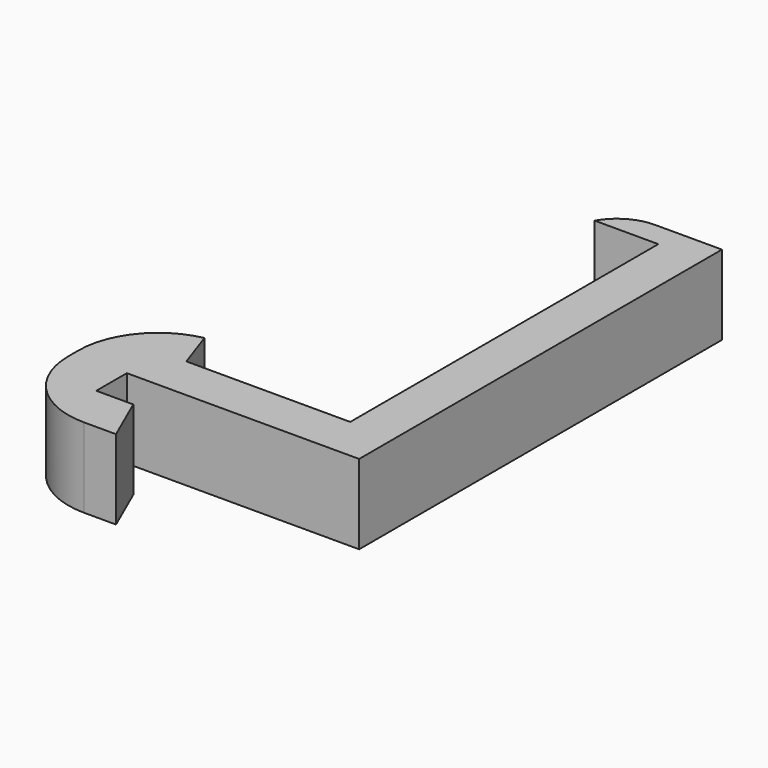
from build123d import *

# Parameters (mm, degrees)
F0_W        = 0.4
F0_H        = 28.4
F1_DEPTH    = 5
F2_T1_DEPTH = 17.9903810568
F3_T1_DEPTH = 29.4948974279
F3_T3_DEPTH = 30


# Not quite as in the source:
# - a fillet or chamfer that OpenCascade refuses, or shapes differently, is made with other operations: its cross-section is extruded or revolved along the edge and cut away or added


with BuildPart() as f1:
    # F0 (on Top) → F1 (new body)
    with BuildSketch(Plane.XY):
        Polygon((-17.5608190332, -5.5), (-10.5608190332, -5.5), (-11.8766345504, -2.5), (-14.2008190332, -2.5), (-14.2008190332, -0.1), (-14.2008190332, 0), (0, 0), (0, 28.4), (-6.4, 28.4), (-6.4, 26.9), (-2.4, 26.9), (-2.4, 2.7), (-12.7, 2.7), (-13.5608190332, 5.2), (-17.5608190332, 5.2), align=None)
        Polygon((-14.2008190332, 0), (-14.2008190332, -0.1), (0.4, -0.1), (0.4, 0), (0, 0), align=None)
        with Locations((0.2, 14.2)):
            Rectangle(F0_W, F0_H)
    extrude(amount=F1_DEPTH)

    # F2: fillet of radius 3 on 1 edges, made by hand

    # F2_s2 → F2_t1 (cut)
    with BuildSketch(Plane.XY.offset(-6.4951905284)):
        with BuildLine():
            ThreePointArc((-3.8019237886, 28.4), (-5.3019237886, 27.9980762114), (-6.4, 26.9))
            Line((-6.4, 26.9), (-6.4, 28.4))
            Line((-6.4, 28.4), (-3.8019237886, 28.4))
        make_face()
    extrude(amount=F2_T1_DEPTH, mode=Mode.SUBTRACT)

    # F3: fillet of radius 5 on 2 edges, made by hand

    # F3_s2 → F3_t1 (cut)
    with BuildSketch(Plane.XY.offset(-12.2474487139)):
        with BuildLine():
            ThreePointArc((-17.5608190332, 0.3010205144), (-16.4338023794, 3.4632981746), (-13.5608190332, 5.2))
            Line((-13.5608190332, 5.2), (-17.5608190332, 5.2))
            Line((-17.5608190332, 5.2), (-17.5608190332, 0.3010205144))
        make_face()
    extrude(amount=F3_T1_DEPTH, mode=Mode.SUBTRACT)

    # F3_s4 → F3_t3 (cut)
    with BuildSketch(Plane.XY.offset(-12.5)):
        with BuildLine():
            ThreePointArc((-17.5608190332, -0.5), (-16.0963529392, -4.0355339059), (-12.5608190332, -5.5))
            Line((-12.5608190332, -5.5), (-17.5608190332, -5.5))
            Line((-17.5608190332, -5.5), (-17.5608190332, -0.5))
        make_face()
    extrude(amount=F3_T3_DEPTH, mode=Mode.SUBTRACT)


solid = f1.part
